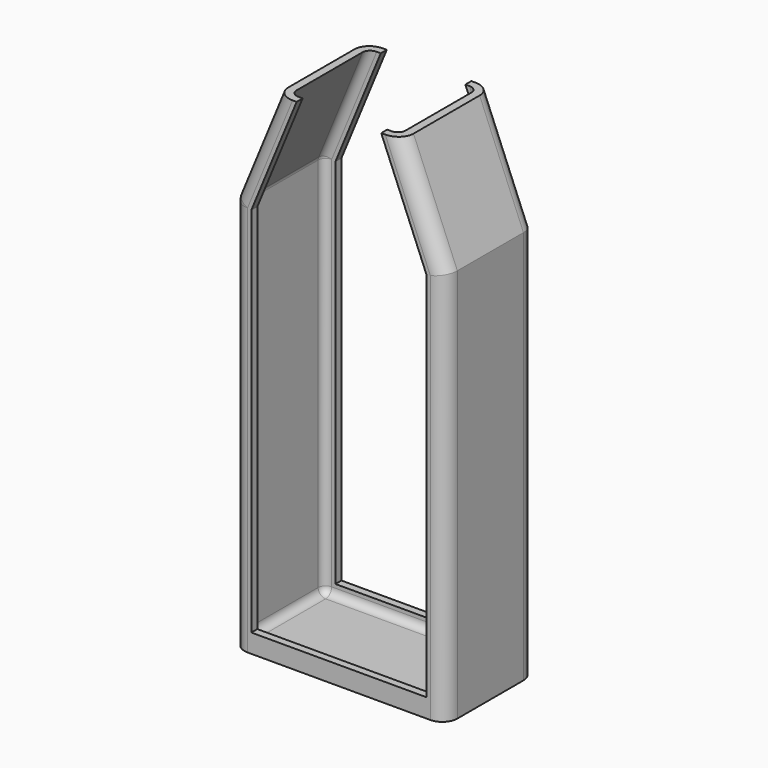
from build123d import *

# Parameters (mm, degrees)
F0_W       = 34
F0_H       = 18
F1_DEPTH   = 80
F2_SIZE2   = 7
F2_SIZE    = 17
F2_2_SIZE2 = 7
F2_2_SIZE  = 17
F3_T       = -1.2
F5_DEPTH   = 18.001
F6_R       = 1.2
F7_R       = 2.4


with BuildPart() as f1:
    # F0 (on Top) → F1 (new body)
    with BuildSketch(Plane.XY):
        Rectangle(F0_W, F0_H)
    extrude(amount=F1_DEPTH)

    # F2
    f2_edges = [f1.edges().sort_by_distance(p)[0] for p in [
        (-17, 0, 80),
    ]]
    f2_side = f1.faces().sort_by_distance((-17, 0, 40))[0]
    chamfer(f2_edges, length=F2_SIZE, length2=F2_SIZE2, reference=f2_side)

    # F2#2
    f2_2_edges = [f1.edges().sort_by_distance(p)[0] for p in [
        (17, 0, 80),
    ]]
    f2_2_side = f1.faces().sort_by_distance((17, 0, 40))[0]
    chamfer(f2_2_edges, length=F2_2_SIZE, length2=F2_2_SIZE2, reference=f2_2_side)

    # F3
    f3_openings = [f1.faces().sort_by_distance(p)[0] for p in [
        (0, 0, 80),
    ]]
    offset(amount=F3_T, openings=f3_openings)

    # F4 (on face) → F5 (cut, through all)
    with BuildSketch(Plane.XZ.offset(9)):
        Polygon((-6.7556277098, 80), (-14, 62.4065244382), (-14, 3), (14, 3), (14, 62.4065244382), (6.7556277098, 80), align=None)
    extrude(amount=-F5_DEPTH, mode=Mode.SUBTRACT)

    # F6
    f6_edges = [f1.edges().sort_by_distance(p)[0] for p in [
        (0, 7.8, 1.2),
        (-15.8, 7.8, 31.981305),
        (-15.8, -7.8, 31.981305),
        (15.8, -7.8, 31.981305),
        (15.8, 0, 1.2),
        (15.8, 7.8, 31.981305),
        (-15.8, 0, 1.2),
        (0, -7.8, 1.2),
        (-12.251126, -7.8, 71.381305),
        (12.251126, -7.8, 71.381305),
        (15.8, 0, 62.76261),
        (12.251126, 7.8, 71.381305),
        (-12.251126, 7.8, 71.381305),
        (-15.8, 0, 62.76261),
    ]]
    fillet(f6_edges, radius=F6_R)

    # F7
    f7_edges = [f1.edges().sort_by_distance(p)[0] for p in [
        (-17, 9, 31.5),
        (17, 9, 31.5),
        (-17, -9, 31.5),
        (-13.5, 9, 71.5),
        (-17, 0, 63),
        (-13.5, -9, 71.5),
        (13.5, -9, 71.5),
        (17, -9, 31.5),
        (13.5, 9, 71.5),
    ]]
    fillet(f7_edges, radius=F7_R)


solid = f1.part
